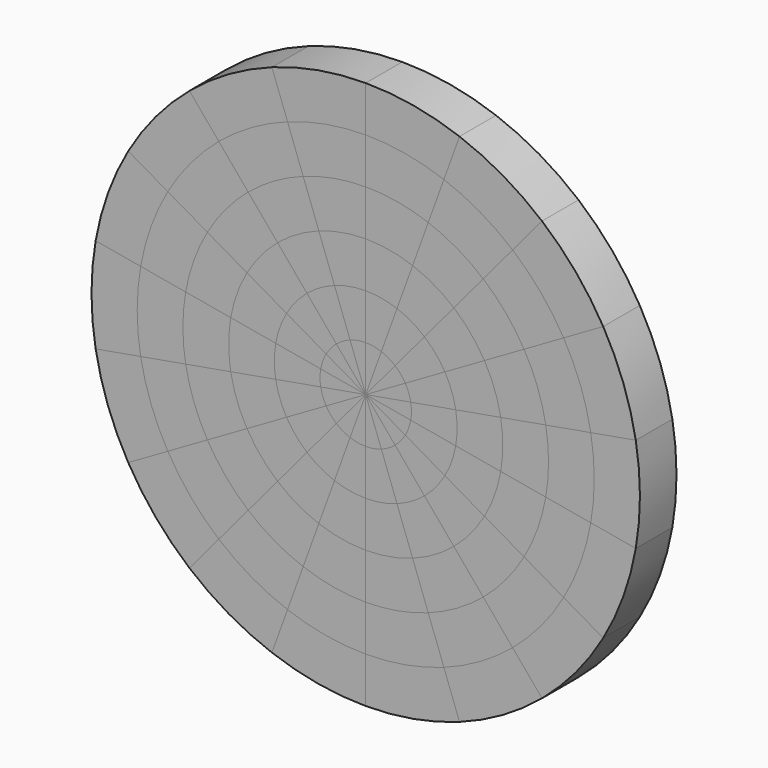
from build123d import *

# Parameters (mm, degrees)
F1_DEPTH = 25
F2_DEPTH = 25
F3_COUNT = 18


with BuildPart() as f1:
    # F0 (on Front) → F1 (new body)
    with BuildSketch(Plane.XZ):
        with BuildLine():
            Line((0, 125), (0, 150))
            ThreePointArc((0, 150), (-26.04722665, 147.7211629518), (-51.3030214989, 140.9538931179))
            Line((-51.3030214989, 140.9538931179), (-42.7525179157, 117.4615775982))
            ThreePointArc((-42.7525179157, 117.4615775982), (-21.7060222084, 123.1009691265), (0, 125))
        make_face()
    extrude(amount=F1_DEPTH)


with BuildPart() as f1b:
    # F0 (on Front) → F1, piece 2 (new body)
    with BuildSketch(Plane.XZ):
        with BuildLine():
            Line((0, 75), (0, 100))
            ThreePointArc((0, 100), (-17.3648177667, 98.4807753012), (-34.2020143326, 93.9692620786))
            Line((-34.2020143326, 93.9692620786), (-25.6515107494, 70.4769465589))
            ThreePointArc((-25.6515107494, 70.4769465589), (-13.023613325, 73.8605814759), (0, 75))
        make_face()
    extrude(amount=F1_DEPTH)


with BuildPart() as f1c:
    # F0 (on Front) → F1, piece 3 (new body)
    with BuildSketch(Plane.XZ):
        with BuildLine():
            Line((0, 25), (0, 50))
            ThreePointArc((0, 50), (-8.6824088833, 49.2403876506), (-17.1010071663, 46.9846310393))
            Line((-17.1010071663, 46.9846310393), (-8.5505035831, 23.4923155196))
            ThreePointArc((-8.5505035831, 23.4923155196), (-4.3412044417, 24.6201938253), (0, 25))
        make_face()
    extrude(amount=F1_DEPTH)


with BuildPart() as f2:
    # F0 (on Front) → F2 (new body)
    with BuildSketch(Plane.XZ):
        with BuildLine():
            Line((0, 100), (0, 125))
            ThreePointArc((0, 125), (-21.7060222084, 123.1009691265), (-42.7525179157, 117.4615775982))
            Line((-42.7525179157, 117.4615775982), (-34.2020143326, 93.9692620786))
            ThreePointArc((-34.2020143326, 93.9692620786), (-17.3648177667, 98.4807753012), (0, 100))
        make_face()
    extrude(amount=F2_DEPTH)


with BuildPart() as f2b:
    # F0 (on Front) → F2, piece 2 (new body)
    with BuildSketch(Plane.XZ):
        with BuildLine():
            Line((0, 50), (0, 75))
            ThreePointArc((0, 75), (-13.023613325, 73.8605814759), (-25.6515107494, 70.4769465589))
            Line((-25.6515107494, 70.4769465589), (-17.1010071663, 46.9846310393))
            ThreePointArc((-17.1010071663, 46.9846310393), (-8.6824088833, 49.2403876506), (0, 50))
        make_face()
    extrude(amount=F2_DEPTH)


with BuildPart() as f2c:
    # F0 (on Front) → F2, piece 3 (new body)
    with BuildSketch(Plane.XZ):
        with BuildLine():
            Line((0, 0), (0, 25))
            ThreePointArc((0, 25), (-4.3412044417, 24.6201938253), (-8.5505035831, 23.4923155196))
            Line((-8.5505035831, 23.4923155196), (0, 0))
        make_face()
    extrude(amount=F2_DEPTH)


with BuildPart() as f3_1:
    # F3: instance of F1
    add(f1.part.rotate(Axis((0, -12.5, 0), (0, 1, 0)), 1 * 360 / F3_COUNT))


with BuildPart() as f3_2:
    # F3: instance of F1
    add(f1.part.rotate(Axis((0, -12.5, 0), (0, 1, 0)), 2 * 360 / F3_COUNT))


with BuildPart() as f3_3:
    # F3: instance of F1
    add(f1.part.rotate(Axis((0, -12.5, 0), (0, 1, 0)), 3 * 360 / F3_COUNT))


with BuildPart() as f3_4:
    # F3: instance of F1
    add(f1.part.rotate(Axis((0, -12.5, 0), (0, 1, 0)), 4 * 360 / F3_COUNT))


with BuildPart() as f3_5:
    # F3: instance of F1
    add(f1.part.rotate(Axis((0, -12.5, 0), (0, 1, 0)), 5 * 360 / F3_COUNT))


with BuildPart() as f3_6:
    # F3: instance of F1
    add(f1.part.rotate(Axis((0, -12.5, 0), (0, 1, 0)), 6 * 360 / F3_COUNT))


with BuildPart() as f3_7:
    # F3: instance of F1
    add(f1.part.rotate(Axis((0, -12.5, 0), (0, 1, 0)), 7 * 360 / F3_COUNT))


with BuildPart() as f3_8:
    # F3: instance of F1
    add(f1.part.rotate(Axis((0, -12.5, 0), (0, 1, 0)), 8 * 360 / F3_COUNT))


with BuildPart() as f3_9:
    # F3: instance of F1
    add(f1.part.rotate(Axis((0, -12.5, 0), (0, 1, 0)), 9 * 360 / F3_COUNT))


with BuildPart() as f3_10:
    # F3: instance of F1
    add(f1.part.rotate(Axis((0, -12.5, 0), (0, 1, 0)), 10 * 360 / F3_COUNT))


with BuildPart() as f3_11:
    # F3: instance of F1
    add(f1.part.rotate(Axis((0, -12.5, 0), (0, 1, 0)), 11 * 360 / F3_COUNT))


with BuildPart() as f3_12:
    # F3: instance of F1
    add(f1.part.rotate(Axis((0, -12.5, 0), (0, 1, 0)), 12 * 360 / F3_COUNT))


with BuildPart() as f3_13:
    # F3: instance of F1
    add(f1.part.rotate(Axis((0, -12.5, 0), (0, 1, 0)), 13 * 360 / F3_COUNT))


with BuildPart() as f3_14:
    # F3: instance of F1
    add(f1.part.rotate(Axis((0, -12.5, 0), (0, 1, 0)), 14 * 360 / F3_COUNT))


with BuildPart() as f3_15:
    # F3: instance of F1
    add(f1.part.rotate(Axis((0, -12.5, 0), (0, 1, 0)), 15 * 360 / F3_COUNT))


with BuildPart() as f3_16:
    # F3: instance of F1
    add(f1.part.rotate(Axis((0, -12.5, 0), (0, 1, 0)), 16 * 360 / F3_COUNT))


with BuildPart() as f3_17:
    # F3: instance of F1
    add(f1.part.rotate(Axis((0, -12.5, 0), (0, 1, 0)), 17 * 360 / F3_COUNT))


with BuildPart() as f3_18:
    # F3: instance of F2
    add(f2.part.rotate(Axis((0, -12.5, 0), (0, 1, 0)), 1 * 360 / F3_COUNT))


with BuildPart() as f3_19:
    # F3: instance of F2
    add(f2.part.rotate(Axis((0, -12.5, 0), (0, 1, 0)), 2 * 360 / F3_COUNT))


with BuildPart() as f3_20:
    # F3: instance of F2
    add(f2.part.rotate(Axis((0, -12.5, 0), (0, 1, 0)), 3 * 360 / F3_COUNT))


with BuildPart() as f3_21:
    # F3: instance of F2
    add(f2.part.rotate(Axis((0, -12.5, 0), (0, 1, 0)), 4 * 360 / F3_COUNT))


with BuildPart() as f3_22:
    # F3: instance of F2
    add(f2.part.rotate(Axis((0, -12.5, 0), (0, 1, 0)), 5 * 360 / F3_COUNT))


with BuildPart() as f3_23:
    # F3: instance of F2
    add(f2.part.rotate(Axis((0, -12.5, 0), (0, 1, 0)), 6 * 360 / F3_COUNT))


with BuildPart() as f3_24:
    # F3: instance of F2
    add(f2.part.rotate(Axis((0, -12.5, 0), (0, 1, 0)), 7 * 360 / F3_COUNT))


with BuildPart() as f3_25:
    # F3: instance of F2
    add(f2.part.rotate(Axis((0, -12.5, 0), (0, 1, 0)), 8 * 360 / F3_COUNT))


with BuildPart() as f3_26:
    # F3: instance of F2
    add(f2.part.rotate(Axis((0, -12.5, 0), (0, 1, 0)), 9 * 360 / F3_COUNT))


with BuildPart() as f3_27:
    # F3: instance of F2
    add(f2.part.rotate(Axis((0, -12.5, 0), (0, 1, 0)), 10 * 360 / F3_COUNT))


with BuildPart() as f3_28:
    # F3: instance of F2
    add(f2.part.rotate(Axis((0, -12.5, 0), (0, 1, 0)), 11 * 360 / F3_COUNT))


with BuildPart() as f3_29:
    # F3: instance of F2
    add(f2.part.rotate(Axis((0, -12.5, 0), (0, 1, 0)), 12 * 360 / F3_COUNT))


with BuildPart() as f3_30:
    # F3: instance of F2
    add(f2.part.rotate(Axis((0, -12.5, 0), (0, 1, 0)), 13 * 360 / F3_COUNT))


with BuildPart() as f3_31:
    # F3: instance of F2
    add(f2.part.rotate(Axis((0, -12.5, 0), (0, 1, 0)), 14 * 360 / F3_COUNT))


with BuildPart() as f3_32:
    # F3: instance of F2
    add(f2.part.rotate(Axis((0, -12.5, 0), (0, 1, 0)), 15 * 360 / F3_COUNT))


with BuildPart() as f3_33:
    # F3: instance of F2
    add(f2.part.rotate(Axis((0, -12.5, 0), (0, 1, 0)), 16 * 360 / F3_COUNT))


with BuildPart() as f3_34:
    # F3: instance of F2
    add(f2.part.rotate(Axis((0, -12.5, 0), (0, 1, 0)), 17 * 360 / F3_COUNT))


with BuildPart() as f3_35:
    # F3: instance of F1b
    add(f1b.part.rotate(Axis((0, -12.5, 0), (0, 1, 0)), 1 * 360 / F3_COUNT))


with BuildPart() as f3_36:
    # F3: instance of F1b
    add(f1b.part.rotate(Axis((0, -12.5, 0), (0, 1, 0)), 2 * 360 / F3_COUNT))


with BuildPart() as f3_37:
    # F3: instance of F1b
    add(f1b.part.rotate(Axis((0, -12.5, 0), (0, 1, 0)), 3 * 360 / F3_COUNT))


with BuildPart() as f3_38:
    # F3: instance of F1b
    add(f1b.part.rotate(Axis((0, -12.5, 0), (0, 1, 0)), 4 * 360 / F3_COUNT))


with BuildPart() as f3_39:
    # F3: instance of F1b
    add(f1b.part.rotate(Axis((0, -12.5, 0), (0, 1, 0)), 5 * 360 / F3_COUNT))


with BuildPart() as f3_40:
    # F3: instance of F1b
    add(f1b.part.rotate(Axis((0, -12.5, 0), (0, 1, 0)), 6 * 360 / F3_COUNT))


with BuildPart() as f3_41:
    # F3: instance of F1b
    add(f1b.part.rotate(Axis((0, -12.5, 0), (0, 1, 0)), 7 * 360 / F3_COUNT))


with BuildPart() as f3_42:
    # F3: instance of F1b
    add(f1b.part.rotate(Axis((0, -12.5, 0), (0, 1, 0)), 8 * 360 / F3_COUNT))


with BuildPart() as f3_43:
    # F3: instance of F1b
    add(f1b.part.rotate(Axis((0, -12.5, 0), (0, 1, 0)), 9 * 360 / F3_COUNT))


with BuildPart() as f3_44:
    # F3: instance of F1b
    add(f1b.part.rotate(Axis((0, -12.5, 0), (0, 1, 0)), 10 * 360 / F3_COUNT))


with BuildPart() as f3_45:
    # F3: instance of F1b
    add(f1b.part.rotate(Axis((0, -12.5, 0), (0, 1, 0)), 11 * 360 / F3_COUNT))


with BuildPart() as f3_46:
    # F3: instance of F1b
    add(f1b.part.rotate(Axis((0, -12.5, 0), (0, 1, 0)), 12 * 360 / F3_COUNT))


with BuildPart() as f3_47:
    # F3: instance of F1b
    add(f1b.part.rotate(Axis((0, -12.5, 0), (0, 1, 0)), 13 * 360 / F3_COUNT))


with BuildPart() as f3_48:
    # F3: instance of F1b
    add(f1b.part.rotate(Axis((0, -12.5, 0), (0, 1, 0)), 14 * 360 / F3_COUNT))


with BuildPart() as f3_49:
    # F3: instance of F1b
    add(f1b.part.rotate(Axis((0, -12.5, 0), (0, 1, 0)), 15 * 360 / F3_COUNT))


with BuildPart() as f3_50:
    # F3: instance of F1b
    add(f1b.part.rotate(Axis((0, -12.5, 0), (0, 1, 0)), 16 * 360 / F3_COUNT))


with BuildPart() as f3_51:
    # F3: instance of F1b
    add(f1b.part.rotate(Axis((0, -12.5, 0), (0, 1, 0)), 17 * 360 / F3_COUNT))


with BuildPart() as f3_52:
    # F3: instance of F2b
    add(f2b.part.rotate(Axis((0, -12.5, 0), (0, 1, 0)), 1 * 360 / F3_COUNT))


with BuildPart() as f3_53:
    # F3: instance of F2b
    add(f2b.part.rotate(Axis((0, -12.5, 0), (0, 1, 0)), 2 * 360 / F3_COUNT))


with BuildPart() as f3_54:
    # F3: instance of F2b
    add(f2b.part.rotate(Axis((0, -12.5, 0), (0, 1, 0)), 3 * 360 / F3_COUNT))


with BuildPart() as f3_55:
    # F3: instance of F2b
    add(f2b.part.rotate(Axis((0, -12.5, 0), (0, 1, 0)), 4 * 360 / F3_COUNT))


with BuildPart() as f3_56:
    # F3: instance of F2b
    add(f2b.part.rotate(Axis((0, -12.5, 0), (0, 1, 0)), 5 * 360 / F3_COUNT))


with BuildPart() as f3_57:
    # F3: instance of F2b
    add(f2b.part.rotate(Axis((0, -12.5, 0), (0, 1, 0)), 6 * 360 / F3_COUNT))


with BuildPart() as f3_58:
    # F3: instance of F2b
    add(f2b.part.rotate(Axis((0, -12.5, 0), (0, 1, 0)), 7 * 360 / F3_COUNT))


with BuildPart() as f3_59:
    # F3: instance of F2b
    add(f2b.part.rotate(Axis((0, -12.5, 0), (0, 1, 0)), 8 * 360 / F3_COUNT))


with BuildPart() as f3_60:
    # F3: instance of F2b
    add(f2b.part.rotate(Axis((0, -12.5, 0), (0, 1, 0)), 9 * 360 / F3_COUNT))


with BuildPart() as f3_61:
    # F3: instance of F2b
    add(f2b.part.rotate(Axis((0, -12.5, 0), (0, 1, 0)), 10 * 360 / F3_COUNT))


with BuildPart() as f3_62:
    # F3: instance of F2b
    add(f2b.part.rotate(Axis((0, -12.5, 0), (0, 1, 0)), 11 * 360 / F3_COUNT))


with BuildPart() as f3_63:
    # F3: instance of F2b
    add(f2b.part.rotate(Axis((0, -12.5, 0), (0, 1, 0)), 12 * 360 / F3_COUNT))


with BuildPart() as f3_64:
    # F3: instance of F2b
    add(f2b.part.rotate(Axis((0, -12.5, 0), (0, 1, 0)), 13 * 360 / F3_COUNT))


with BuildPart() as f3_65:
    # F3: instance of F2b
    add(f2b.part.rotate(Axis((0, -12.5, 0), (0, 1, 0)), 14 * 360 / F3_COUNT))


with BuildPart() as f3_66:
    # F3: instance of F2b
    add(f2b.part.rotate(Axis((0, -12.5, 0), (0, 1, 0)), 15 * 360 / F3_COUNT))


with BuildPart() as f3_67:
    # F3: instance of F2b
    add(f2b.part.rotate(Axis((0, -12.5, 0), (0, 1, 0)), 16 * 360 / F3_COUNT))


with BuildPart() as f3_68:
    # F3: instance of F2b
    add(f2b.part.rotate(Axis((0, -12.5, 0), (0, 1, 0)), 17 * 360 / F3_COUNT))


with BuildPart() as f3_69:
    # F3: instance of F1c
    add(f1c.part.rotate(Axis((0, -12.5, 0), (0, 1, 0)), 1 * 360 / F3_COUNT))


with BuildPart() as f3_70:
    # F3: instance of F1c
    add(f1c.part.rotate(Axis((0, -12.5, 0), (0, 1, 0)), 2 * 360 / F3_COUNT))


with BuildPart() as f3_71:
    # F3: instance of F1c
    add(f1c.part.rotate(Axis((0, -12.5, 0), (0, 1, 0)), 3 * 360 / F3_COUNT))


with BuildPart() as f3_72:
    # F3: instance of F1c
    add(f1c.part.rotate(Axis((0, -12.5, 0), (0, 1, 0)), 4 * 360 / F3_COUNT))


with BuildPart() as f3_73:
    # F3: instance of F1c
    add(f1c.part.rotate(Axis((0, -12.5, 0), (0, 1, 0)), 5 * 360 / F3_COUNT))


with BuildPart() as f3_74:
    # F3: instance of F1c
    add(f1c.part.rotate(Axis((0, -12.5, 0), (0, 1, 0)), 6 * 360 / F3_COUNT))


with BuildPart() as f3_75:
    # F3: instance of F1c
    add(f1c.part.rotate(Axis((0, -12.5, 0), (0, 1, 0)), 7 * 360 / F3_COUNT))


with BuildPart() as f3_76:
    # F3: instance of F1c
    add(f1c.part.rotate(Axis((0, -12.5, 0), (0, 1, 0)), 8 * 360 / F3_COUNT))


with BuildPart() as f3_77:
    # F3: instance of F1c
    add(f1c.part.rotate(Axis((0, -12.5, 0), (0, 1, 0)), 9 * 360 / F3_COUNT))


with BuildPart() as f3_78:
    # F3: instance of F1c
    add(f1c.part.rotate(Axis((0, -12.5, 0), (0, 1, 0)), 10 * 360 / F3_COUNT))


with BuildPart() as f3_79:
    # F3: instance of F1c
    add(f1c.part.rotate(Axis((0, -12.5, 0), (0, 1, 0)), 11 * 360 / F3_COUNT))


with BuildPart() as f3_80:
    # F3: instance of F1c
    add(f1c.part.rotate(Axis((0, -12.5, 0), (0, 1, 0)), 12 * 360 / F3_COUNT))


with BuildPart() as f3_81:
    # F3: instance of F1c
    add(f1c.part.rotate(Axis((0, -12.5, 0), (0, 1, 0)), 13 * 360 / F3_COUNT))


with BuildPart() as f3_82:
    # F3: instance of F1c
    add(f1c.part.rotate(Axis((0, -12.5, 0), (0, 1, 0)), 14 * 360 / F3_COUNT))


with BuildPart() as f3_83:
    # F3: instance of F1c
    add(f1c.part.rotate(Axis((0, -12.5, 0), (0, 1, 0)), 15 * 360 / F3_COUNT))


with BuildPart() as f3_84:
    # F3: instance of F1c
    add(f1c.part.rotate(Axis((0, -12.5, 0), (0, 1, 0)), 16 * 360 / F3_COUNT))


with BuildPart() as f3_85:
    # F3: instance of F1c
    add(f1c.part.rotate(Axis((0, -12.5, 0), (0, 1, 0)), 17 * 360 / F3_COUNT))


with BuildPart() as f3_86:
    # F3: instance of F2c
    add(f2c.part.rotate(Axis((0, -12.5, 0), (0, 1, 0)), 1 * 360 / F3_COUNT))


with BuildPart() as f3_87:
    # F3: instance of F2c
    add(f2c.part.rotate(Axis((0, -12.5, 0), (0, 1, 0)), 2 * 360 / F3_COUNT))


with BuildPart() as f3_88:
    # F3: instance of F2c
    add(f2c.part.rotate(Axis((0, -12.5, 0), (0, 1, 0)), 3 * 360 / F3_COUNT))


with BuildPart() as f3_89:
    # F3: instance of F2c
    add(f2c.part.rotate(Axis((0, -12.5, 0), (0, 1, 0)), 4 * 360 / F3_COUNT))


with BuildPart() as f3_90:
    # F3: instance of F2c
    add(f2c.part.rotate(Axis((0, -12.5, 0), (0, 1, 0)), 5 * 360 / F3_COUNT))


with BuildPart() as f3_91:
    # F3: instance of F2c
    add(f2c.part.rotate(Axis((0, -12.5, 0), (0, 1, 0)), 6 * 360 / F3_COUNT))


with BuildPart() as f3_92:
    # F3: instance of F2c
    add(f2c.part.rotate(Axis((0, -12.5, 0), (0, 1, 0)), 7 * 360 / F3_COUNT))


with BuildPart() as f3_93:
    # F3: instance of F2c
    add(f2c.part.rotate(Axis((0, -12.5, 0), (0, 1, 0)), 8 * 360 / F3_COUNT))


with BuildPart() as f3_94:
    # F3: instance of F2c
    add(f2c.part.rotate(Axis((0, -12.5, 0), (0, 1, 0)), 9 * 360 / F3_COUNT))


with BuildPart() as f3_95:
    # F3: instance of F2c
    add(f2c.part.rotate(Axis((0, -12.5, 0), (0, 1, 0)), 10 * 360 / F3_COUNT))


with BuildPart() as f3_96:
    # F3: instance of F2c
    add(f2c.part.rotate(Axis((0, -12.5, 0), (0, 1, 0)), 11 * 360 / F3_COUNT))


with BuildPart() as f3_97:
    # F3: instance of F2c
    add(f2c.part.rotate(Axis((0, -12.5, 0), (0, 1, 0)), 12 * 360 / F3_COUNT))


with BuildPart() as f3_98:
    # F3: instance of F2c
    add(f2c.part.rotate(Axis((0, -12.5, 0), (0, 1, 0)), 13 * 360 / F3_COUNT))


with BuildPart() as f3_99:
    # F3: instance of F2c
    add(f2c.part.rotate(Axis((0, -12.5, 0), (0, 1, 0)), 14 * 360 / F3_COUNT))


with BuildPart() as f3_100:
    # F3: instance of F2c
    add(f2c.part.rotate(Axis((0, -12.5, 0), (0, 1, 0)), 15 * 360 / F3_COUNT))


with BuildPart() as f3_101:
    # F3: instance of F2c
    add(f2c.part.rotate(Axis((0, -12.5, 0), (0, 1, 0)), 16 * 360 / F3_COUNT))


with BuildPart() as f3_102:
    # F3: instance of F2c
    add(f2c.part.rotate(Axis((0, -12.5, 0), (0, 1, 0)), 17 * 360 / F3_COUNT))


solid = Compound([f1.part, f1b.part, f1c.part, f2.part, f2b.part, f2c.part, f3_1.part, f3_2.part, f3_3.part, f3_4.part, f3_5.part, f3_6.part, f3_7.part, f3_8.part, f3_9.part, f3_10.part, f3_11.part, f3_12.part, f3_13.part, f3_14.part, f3_15.part, f3_16.part, f3_17.part, f3_18.part, f3_19.part, f3_20.part, f3_21.part, f3_22.part, f3_23.part, f3_24.part, f3_25.part, f3_26.part, f3_27.part, f3_28.part, f3_29.part, f3_30.part, f3_31.part, f3_32.part, f3_33.part, f3_34.part, f3_35.part, f3_36.part, f3_37.part, f3_38.part, f3_39.part, f3_40.part, f3_41.part, f3_42.part, f3_43.part, f3_44.part, f3_45.part, f3_46.part, f3_47.part, f3_48.part, f3_49.part, f3_50.part, f3_51.part, f3_52.part, f3_53.part, f3_54.part, f3_55.part, f3_56.part, f3_57.part, f3_58.part, f3_59.part, f3_60.part, f3_61.part, f3_62.part, f3_63.part, f3_64.part, f3_65.part, f3_66.part, f3_67.part, f3_68.part, f3_69.part, f3_70.part, f3_71.part, f3_72.part, f3_73.part, f3_74.part, f3_75.part, f3_76.part, f3_77.part, f3_78.part, f3_79.part, f3_80.part, f3_81.part, f3_82.part, f3_83.part, f3_84.part, f3_85.part, f3_86.part, f3_87.part, f3_88.part, f3_89.part, f3_90.part, f3_91.part, f3_92.part, f3_93.part, f3_94.part, f3_95.part, f3_96.part, f3_97.part, f3_98.part, f3_99.part, f3_100.part, f3_101.part, f3_102.part])
